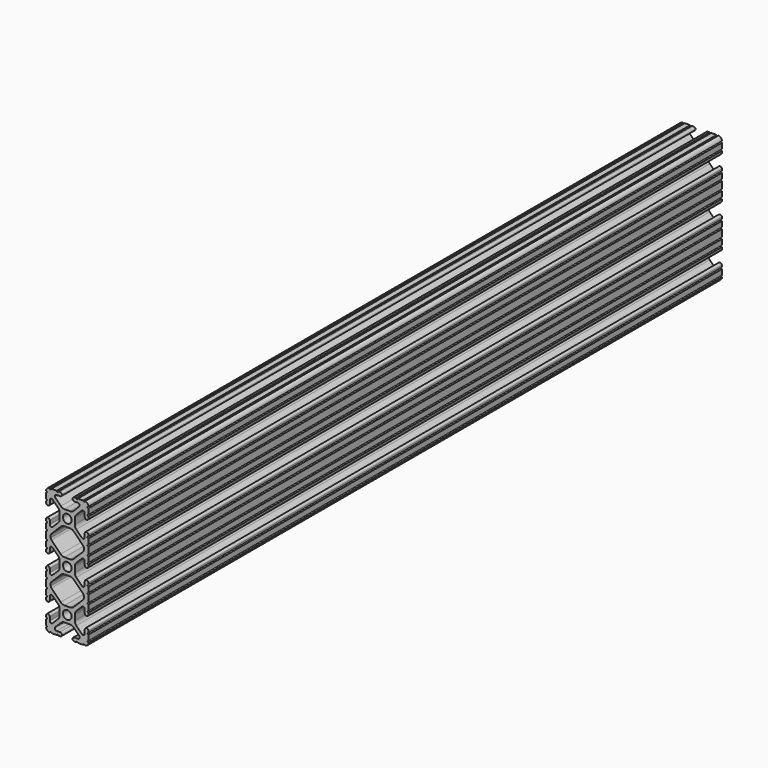
from build123d import *

# Parameters (mm, degrees)
F1_DEPTH = 475


# Not quite as in the source:
# - ends of sketch curves that miss each other by under 0.0002 mm in the source are joined


with BuildPart() as f1:
    # F0 (on Front) → F1 (new body)
    with BuildSketch(Plane.XZ):
        with BuildLine():
            ThreePointArc((-9.5504, 38.1), (-10.0584, 37.592), (-10.5664, 38.1))
            ThreePointArc((-10.5664, 38.1), (-12.0826749161, 37.4826749161), (-12.699997541, 35.9664000298))
            ThreePointArc((-12.699997541, 35.9664000298), (-12.192, 35.4584), (-12.7, 34.9504))
            Line((-12.7, 34.9504), (-12.7, 31.7246))
            ThreePointArc((-12.7, 31.7246), (-12.192, 31.2166), (-12.7, 30.7086))
            Line((-12.7, 30.7086), (-12.7, 29.7023028))
            ThreePointArc((-12.7, 29.7023028), (-11.5951, 28.5974028), (-10.4902, 29.7023028))
            Line((-10.4902, 29.7023028), (-10.4902, 31.8747902))
            ThreePointArc((-10.4902, 31.8747902), (-9.8630063673, 32.813451805), (-8.7557795103, 32.5932106897))
            Line((-8.7557795103, 32.5932106897), (-5.4384448, 29.2758622))
            ThreePointArc((-5.4384448, 29.2758622), (-4.7501824843, 28.2458268978), (-4.5085, 27.030807))
            Line((-4.5085, 27.030807), (-4.5085, 23.769193))
            ThreePointArc((-4.5085, 23.769193), (-4.7501824843, 22.5541731022), (-5.4384359697, 21.5241289697))
            Line((-5.4384359697, 21.5241289697), (-8.7557864, 18.2067962))
            ThreePointArc((-8.7557864, 18.2067962), (-9.8630063673, 17.986548195), (-10.4902, 18.9252098))
            Line((-10.4902, 18.9252098), (-10.4902, 21.0976972))
            ThreePointArc((-10.4902, 21.0976972), (-11.5951, 22.2025972), (-12.7, 21.0976972))
            Line((-12.7, 21.0976972), (-12.7, 20.0914))
            ThreePointArc((-12.7, 20.0914), (-12.192, 19.5834), (-12.7, 19.0754))
            Line((-12.7, 19.0754), (-12.7, 15.8496))
            ThreePointArc((-12.7, 15.8496), (-12.192, 15.3416), (-12.7, 14.8336))
            Line((-12.7, 14.8336), (-12.7, 10.5664))
            ThreePointArc((-12.7, 10.5664), (-12.192, 10.0584), (-12.7, 9.5504))
            Line((-12.7, 9.5504), (-12.7, 6.3246))
            ThreePointArc((-12.7, 6.3246), (-12.192, 5.8166), (-12.7, 5.3086))
            Line((-12.7, 5.3086), (-12.7, 4.3023028))
            ThreePointArc((-12.7, 4.3023028), (-11.5951, 3.1974028), (-10.4902, 4.3023028))
            Line((-10.4902, 4.3023028), (-10.4902, 6.4747902))
            ThreePointArc((-10.4902, 6.4747902), (-9.8630063673, 7.413451805), (-8.7557795103, 7.1932106897))
            Line((-8.7557795103, 7.1932106897), (-5.4384448, 3.8758622))
            ThreePointArc((-5.4384448, 3.8758622), (-4.7501824843, 2.8458268978), (-4.5085, 1.630807))
            Line((-4.5085, 1.630807), (-4.5085, -1.630807))
            ThreePointArc((-4.5085, -1.630807), (-4.7501824843, -2.8458268978), (-5.4384359697, -3.8758710303))
            Line((-5.4384359697, -3.8758710303), (-8.7557864, -7.1932038))
            ThreePointArc((-8.7557864, -7.1932038), (-9.8630063673, -7.413451805), (-10.4902, -6.4747902))
            Line((-10.4902, -6.4747902), (-10.4902, -4.3023028))
            ThreePointArc((-10.4902, -4.3023028), (-11.5951, -3.1974028), (-12.7, -4.3023028))
            Line((-12.7, -4.3023028), (-12.7, -5.3086))
            ThreePointArc((-12.7, -5.3086), (-12.192, -5.8166), (-12.7, -6.3246))
            Line((-12.7, -6.3246), (-12.7, -9.5504))
            ThreePointArc((-12.7, -9.5504), (-12.192, -10.0584), (-12.7, -10.5664))
            Line((-12.7, -10.5664), (-12.7, -14.8336))
            ThreePointArc((-12.7, -14.8336), (-12.192, -15.3416), (-12.7, -15.8496))
            Line((-12.7, -15.8496), (-12.7, -19.0754))
            ThreePointArc((-12.7, -19.0754), (-12.192, -19.5834), (-12.7, -20.0914))
            Line((-12.7, -20.0914), (-12.7, -21.0976972))
            ThreePointArc((-12.7, -21.0976972), (-11.5951, -22.2025972), (-10.4902, -21.0976972))
            Line((-10.4902, -21.0976972), (-10.4902, -18.9252098))
            ThreePointArc((-10.4902, -18.9252098), (-9.8630063673, -17.986548195), (-8.7557795103, -18.2067893103))
            Line((-8.7557795103, -18.2067893103), (-5.4384448, -21.5241378))
            ThreePointArc((-5.4384448, -21.5241378), (-4.7501824843, -22.5541731022), (-4.5085, -23.769193))
            Line((-4.5085, -23.769193), (-4.5085, -27.030807))
            ThreePointArc((-4.5085, -27.030807), (-4.7501824843, -28.2458268978), (-5.4384359697, -29.2758710303))
            Line((-5.4384359697, -29.2758710303), (-8.7557864, -32.5932038))
            ThreePointArc((-8.7557864, -32.5932038), (-9.8630063673, -32.813451805), (-10.4902, -31.8747902))
            Line((-10.4902, -31.8747902), (-10.4902, -29.7023028))
            ThreePointArc((-10.4902, -29.7023028), (-11.5951, -28.5974028), (-12.7, -29.7023028))
            Line((-12.7, -29.7023028), (-12.7, -30.7086))
            ThreePointArc((-12.7, -30.7086), (-12.192, -31.2166), (-12.7, -31.7246))
            Line((-12.7, -31.7246), (-12.7, -34.9504))
            ThreePointArc((-12.7, -34.9504), (-12.192, -35.4584), (-12.7, -35.9664))
            ThreePointArc((-12.7, -35.9664), (-12.0826749161, -37.4826749161), (-10.5664000298, -38.099997541))
            ThreePointArc((-10.5664000298, -38.099997541), (-10.0584, -37.592), (-9.5504, -38.1))
            Line((-9.5504, -38.1), (-6.3246, -38.1))
            ThreePointArc((-6.3246, -38.1), (-5.8166, -37.592), (-5.3086, -38.1))
            Line((-5.3086, -38.1), (-4.3023028, -38.1))
            ThreePointArc((-4.3023028, -38.1), (-3.1974028, -36.9951), (-4.3023028, -35.8902))
            Line((-4.3023028, -35.8902), (-6.4747902, -35.8902))
            ThreePointArc((-6.4747902, -35.8902), (-7.413451805, -35.2630063673), (-7.1932106897, -34.1557795103))
            Line((-7.1932106897, -34.1557795103), (-3.8758622, -30.8384448))
            ThreePointArc((-3.8758622, -30.8384448), (-2.8458268978, -30.1501824843), (-1.630807, -29.9085))
            Line((-1.630807, -29.9085), (1.630807, -29.9085))
            ThreePointArc((1.630807, -29.9085), (2.8458268978, -30.1501824843), (3.8758710303, -30.8384359697))
            Line((3.8758710303, -30.8384359697), (7.1932038, -34.1557864))
            ThreePointArc((7.1932038, -34.1557864), (7.413451805, -35.2630063673), (6.4747902, -35.8902))
            Line((6.4747902, -35.8902), (4.3023028, -35.8902))
            ThreePointArc((4.3023028, -35.8902), (3.1974028, -36.9951), (4.3023028, -38.1))
            Line((4.3023028, -38.1), (5.3086, -38.1))
            ThreePointArc((5.3086, -38.1), (5.8166, -37.592), (6.3246, -38.1))
            Line((6.3246, -38.1), (9.5504, -38.1))
            ThreePointArc((9.5504, -38.1), (10.0584, -37.592), (10.5664, -38.1))
            ThreePointArc((10.5664, -38.1), (12.0826749161, -37.4826749161), (12.699997541, -35.9664000298))
            ThreePointArc((12.699997541, -35.9664000298), (12.192, -35.4584), (12.7, -34.9504))
            Line((12.7, -34.9504), (12.7, -31.7246))
            ThreePointArc((12.7, -31.7246), (12.192, -31.2166), (12.7, -30.7086))
            Line((12.7, -30.7086), (12.7, -29.7023028))
            ThreePointArc((12.7, -29.7023028), (11.5951, -28.5974028), (10.4902, -29.7023028))
            Line((10.4902, -29.7023028), (10.4902, -31.8747902))
            ThreePointArc((10.4902, -31.8747902), (9.8630063673, -32.813451805), (8.7557795103, -32.5932106897))
            Line((8.7557795103, -32.5932106897), (5.4384448, -29.2758622))
            ThreePointArc((5.4384448, -29.2758622), (4.7501824843, -28.2458268978), (4.5085, -27.030807))
            Line((4.5085, -27.030807), (4.5085, -23.769193))
            ThreePointArc((4.5085, -23.769193), (4.7501824843, -22.5541731022), (5.4384359697, -21.5241289697))
            Line((5.4384359697, -21.5241289697), (8.7557864, -18.2067962))
            ThreePointArc((8.7557864, -18.2067962), (9.8630063673, -17.986548195), (10.4902, -18.9252098))
            Line((10.4902, -18.9252098), (10.4902, -21.0976972))
            ThreePointArc((10.4902, -21.0976972), (11.5951, -22.2025972), (12.7, -21.0976972))
            Line((12.7, -21.0976972), (12.7, -20.0914))
            ThreePointArc((12.7, -20.0914), (12.192, -19.5834), (12.7, -19.0754))
            Line((12.7, -19.0754), (12.7, -15.8496))
            ThreePointArc((12.7, -15.8496), (12.192, -15.3416), (12.7, -14.8336))
            Line((12.7, -14.8336), (12.7, -10.5664))
            ThreePointArc((12.7, -10.5664), (12.192, -10.0584), (12.7, -9.5504))
            Line((12.7, -9.5504), (12.7, -6.3246))
            ThreePointArc((12.7, -6.3246), (12.192, -5.8166), (12.7, -5.3086))
            Line((12.7, -5.3086), (12.7, -4.3023028))
            ThreePointArc((12.7, -4.3023028), (11.5951, -3.1974028), (10.4902, -4.3023028))
            Line((10.4902, -4.3023028), (10.4902, -6.4747902))
            ThreePointArc((10.4902, -6.4747902), (9.8630063673, -7.413451805), (8.7557795103, -7.1932106897))
            Line((8.7557795103, -7.1932106897), (5.4384448, -3.8758622))
            ThreePointArc((5.4384448, -3.8758622), (4.7501824843, -2.8458268978), (4.5085, -1.630807))
            Line((4.5085, -1.630807), (4.5085, 1.630807))
            ThreePointArc((4.5085, 1.630807), (4.7501824843, 2.8458268978), (5.4384359697, 3.8758710303))
            Line((5.4384359697, 3.8758710303), (8.7557864, 7.1932038))
            ThreePointArc((8.7557864, 7.1932038), (9.8630063673, 7.413451805), (10.4902, 6.4747902))
            Line((10.4902, 6.4747902), (10.4902, 4.3023028))
            ThreePointArc((10.4902, 4.3023028), (11.5951, 3.1974028), (12.7, 4.3023028))
            Line((12.7, 4.3023028), (12.7, 5.3086))
            ThreePointArc((12.7, 5.3086), (12.192, 5.8166), (12.7, 6.3246))
            Line((12.7, 6.3246), (12.7, 9.5504))
            ThreePointArc((12.7, 9.5504), (12.192, 10.0584), (12.7, 10.5664))
            Line((12.7, 10.5664), (12.7, 14.8336))
            ThreePointArc((12.7, 14.8336), (12.192, 15.3416), (12.7, 15.8496))
            Line((12.7, 15.8496), (12.7, 19.0754))
            ThreePointArc((12.7, 19.0754), (12.192, 19.5834), (12.7, 20.0914))
            Line((12.7, 20.0914), (12.7, 21.0976972))
            ThreePointArc((12.7, 21.0976972), (11.5951, 22.2025972), (10.4902, 21.0976972))
            Line((10.4902, 21.0976972), (10.4902, 18.9252098))
            ThreePointArc((10.4902, 18.9252098), (9.8630063673, 17.986548195), (8.7557795103, 18.2067893103))
            Line((8.7557795103, 18.2067893103), (5.4384448, 21.5241378))
            ThreePointArc((5.4384448, 21.5241378), (4.7501824843, 22.5541731022), (4.5085, 23.769193))
            Line((4.5085, 23.769193), (4.5085, 27.030807))
            ThreePointArc((4.5085, 27.030807), (4.7501824843, 28.2458268978), (5.4384359697, 29.2758710303))
            Line((5.4384359697, 29.2758710303), (8.7557864, 32.5932038))
            ThreePointArc((8.7557864, 32.5932038), (9.8630063673, 32.813451805), (10.4902, 31.8747902))
            Line((10.4902, 31.8747902), (10.4902, 29.7023028))
            ThreePointArc((10.4902, 29.7023028), (11.5951, 28.5974028), (12.7, 29.7023028))
            Line((12.7, 29.7023028), (12.7, 30.7086))
            ThreePointArc((12.7, 30.7086), (12.192, 31.2166), (12.7, 31.7246))
            Line((12.7, 31.7246), (12.7, 34.9504))
            ThreePointArc((12.7, 34.9504), (12.192, 35.4584), (12.7, 35.9664))
            ThreePointArc((12.7, 35.9664), (12.0826749161, 37.4826749161), (10.5664000298, 38.099997541))
            ThreePointArc((10.5664000298, 38.099997541), (10.0584, 37.592), (9.5504, 38.1))
            Line((9.5504, 38.1), (6.3246, 38.1))
            ThreePointArc((6.3246, 38.1), (5.8166, 37.592), (5.3086, 38.1))
            Line((5.3086, 38.1), (4.3023028, 38.1))
            ThreePointArc((4.3023028, 38.1), (3.1974028, 36.9951), (4.3023028, 35.8902))
            Line((4.3023028, 35.8902), (6.4747902, 35.8902))
            ThreePointArc((6.4747902, 35.8902), (7.413451805, 35.2630063673), (7.1932106897, 34.1557795103))
            Line((7.1932106897, 34.1557795103), (3.8758622, 30.8384448))
            ThreePointArc((3.8758622, 30.8384448), (2.8458268978, 30.1501824843), (1.630807, 29.9085))
            Line((1.630807, 29.9085), (-1.630807, 29.9085))
            ThreePointArc((-1.630807, 29.9085), (-2.8458268978, 30.1501824843), (-3.8758710303, 30.8384359697))
            Line((-3.8758710303, 30.8384359697), (-7.1932038, 34.1557864))
            ThreePointArc((-7.1932038, 34.1557864), (-7.413451805, 35.2630063673), (-6.4747902, 35.8902))
            Line((-6.4747902, 35.8902), (-4.3023028, 35.8902))
            ThreePointArc((-4.3023028, 35.8902), (-3.1974028, 36.9951), (-4.3023028, 38.1))
            Line((-4.3023028, 38.1), (-5.3086, 38.1))
            ThreePointArc((-5.3086, 38.1), (-5.8166, 37.592), (-6.3246, 38.1))
            Line((-6.3246, 38.1), (-9.5504, 38.1))
        make_face()
        with BuildLine():
            ThreePointArc((-2.6035, -25.4), (0, -22.7965), (2.6035, -25.4))
            ThreePointArc((2.6035, -25.4), (0, -28.0035), (-2.6035, -25.4))
        make_face(mode=Mode.SUBTRACT)
        with BuildLine():
            Line((-9.4701614, -11.0327186), (-3.8758622, -5.4384448))
            ThreePointArc((-3.8758622, -5.4384448), (-2.8458268978, -4.7501824843), (-1.630807, -4.5085))
            Line((-1.630807, -4.5085), (1.630807, -4.5085))
            ThreePointArc((1.630807, -4.5085), (2.8458268978, -4.7501824843), (3.8758710303, -5.4384359697))
            Line((3.8758710303, -5.4384359697), (9.4701614, -11.0327186))
            ThreePointArc((9.4701614, -11.0327186), (9.8115254878, -11.5436301307), (9.9314, -12.14628))
            Line((9.9314, -12.14628), (9.9314, -13.25372))
            ThreePointArc((9.9314, -13.25372), (9.8115254878, -13.8563698693), (9.470151759, -14.367271759))
            Line((9.470151759, -14.367271759), (3.8758622, -19.9615552))
            ThreePointArc((3.8758622, -19.9615552), (2.8458268978, -20.6498175157), (1.630807, -20.8915))
            Line((1.630807, -20.8915), (-1.630807, -20.8915))
            ThreePointArc((-1.630807, -20.8915), (-2.8458268978, -20.6498175157), (-3.8758710303, -19.9615640303))
            Line((-3.8758710303, -19.9615640303), (-9.4701614, -14.3672814))
            ThreePointArc((-9.4701614, -14.3672814), (-9.8115254878, -13.8563698693), (-9.9314, -13.25372))
            Line((-9.9314, -13.25372), (-9.9314, -12.14628))
            ThreePointArc((-9.9314, -12.14628), (-9.8115254878, -11.5436301307), (-9.4701614, -11.0327186))
        make_face(mode=Mode.SUBTRACT)
        with BuildLine():
            ThreePointArc((-2.6035, 0), (0, 2.6035), (2.6035, 0))
            ThreePointArc((2.6035, 0), (0, -2.6035), (-2.6035, 0))
        make_face(mode=Mode.SUBTRACT)
        with BuildLine():
            Line((-9.4701614, 14.3672814), (-3.8758622, 19.9615552))
            ThreePointArc((-3.8758622, 19.9615552), (-2.8458268978, 20.6498175157), (-1.630807, 20.8915))
            Line((-1.630807, 20.8915), (1.630807, 20.8915))
            ThreePointArc((1.630807, 20.8915), (2.8458268978, 20.6498175157), (3.8758710303, 19.9615640303))
            Line((3.8758710303, 19.9615640303), (9.4701614, 14.3672814))
            ThreePointArc((9.4701614, 14.3672814), (9.8115254878, 13.8563698693), (9.9314, 13.25372))
            Line((9.9314, 13.25372), (9.9314, 12.14628))
            ThreePointArc((9.9314, 12.14628), (9.8115254878, 11.5436301307), (9.470151759, 11.032728241))
            Line((9.470151759, 11.032728241), (3.8758622, 5.4384448))
            ThreePointArc((3.8758622, 5.4384448), (2.8458268978, 4.7501824843), (1.630807, 4.5085))
            Line((1.630807, 4.5085), (-1.630807, 4.5085))
            ThreePointArc((-1.630807, 4.5085), (-2.8458268978, 4.7501824843), (-3.8758710303, 5.4384359697))
            Line((-3.8758710303, 5.4384359697), (-9.4701614, 11.0327186))
            ThreePointArc((-9.4701614, 11.0327186), (-9.8115254878, 11.5436301307), (-9.9314, 12.14628))
            Line((-9.9314, 12.14628), (-9.9314, 13.25372))
            ThreePointArc((-9.9314, 13.25372), (-9.8115254878, 13.8563698693), (-9.4701614, 14.3672814))
        make_face(mode=Mode.SUBTRACT)
        with BuildLine():
            ThreePointArc((-2.6035, 25.4), (0, 28.0035), (2.6035, 25.4))
            ThreePointArc((2.6035, 25.4), (0, 22.7965), (-2.6035, 25.4))
        make_face(mode=Mode.SUBTRACT)
    extrude(amount=F1_DEPTH)


solid = f1.part
